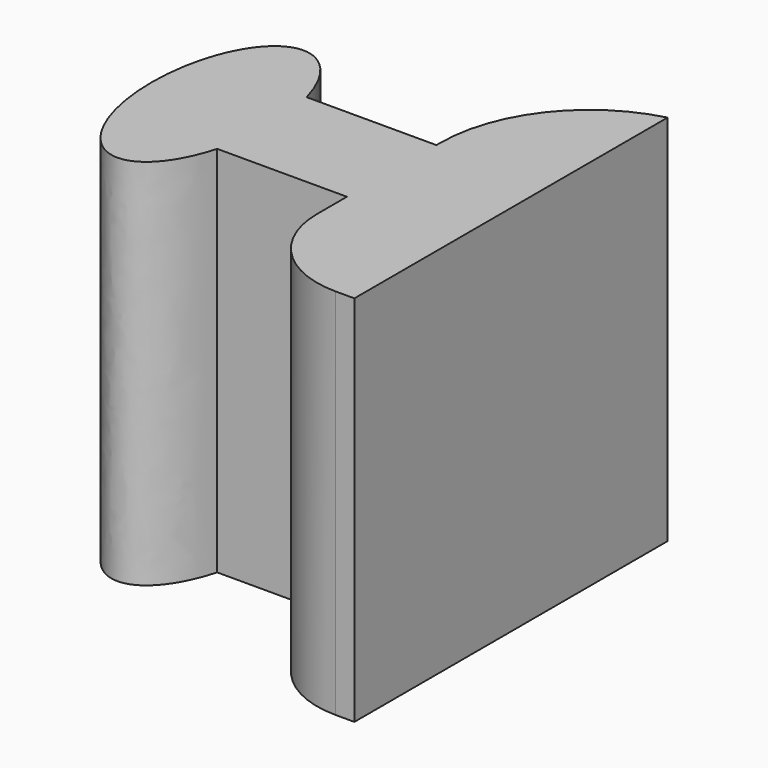
from build123d import *

# Parameters (mm, degrees)
F1_DEPTH    = 10
F2_DEPTH    = 10
F3_T1_DEPTH = 29.364916731
F4_R        = 2.5


# Not quite as in the source:
# - a fillet or chamfer that OpenCascade refuses, or shapes differently, is made with other operations: its cross-section is extruded or revolved along the edge and cut away or added


with BuildPart() as f1:
    # F0 (on Top) → F1 (new body)
    with BuildSketch(Plane.XY):
        with BuildLine():
            Line((0, -5.25), (0, 0))
            Line((0, 0), (0, 5.25))
            Line((0, 5.25), (-3, 5.25))
            Line((-3, 5.25), (-3, 1.25))
            Line((-3, 1.25), (-6.479551384, 1.25))
            add(Edge.make_bspline(
                [(-6.479551384, -1.75), (-6.0631503018, -0.25), (-6.479551384, 1.25)],
                knots=[1.0687204508, 1.0687204508, 1.0687204508, 2.0728722028, 2.0728722028, 2.0728722028], degree=2, weights=[1, 0.8765854438, 1]))
            Line((-6.479551384, -1.75), (-3, -1.75))
            Line((-3, -1.75), (-3, -5.25))
            Line((-3, -5.25), (0, -5.25))
        make_face()
    extrude(amount=F1_DEPTH)

    # F0 (on Top) → F2 (join)
    with BuildSketch(Plane.XY):
        with BuildLine():
            add(Edge.make_bspline(
                [(-6.479551384, -1.75), (-6.0631503018, -0.25), (-6.479551384, 1.25)],
                knots=[1.0687204508, 1.0687204508, 1.0687204508, 2.0728722028, 2.0728722028, 2.0728722028], degree=2, weights=[1, 0.8765854438, 1]))
            add(Edge.make_bspline(
                [(-6.479551384, 1.25), (-7.8097391813, 6.0417303318), (-9.2174427731, 1.3374114859), (-10.6251463649, -3.36690736), (-7.8610982746, -3.36690736)],
                knots=[2.0728722028, 2.0728722028, 2.0728722028, 4.178028755, 4.178028755, 6.2831853072, 6.2831853072, 6.2831853072], degree=2, weights=[1, 0.49533294, 1, 0.49533294, 1]))
            add(Edge.make_bspline(
                [(-7.8610982746, -3.36690736), (-6.9284060337, -3.36690736), (-6.479551384, -1.75)],
                knots=[0, 0, 0, 1.0687204508, 1.0687204508, 1.0687204508], degree=2, weights=[1, 0.8605946365, 1]))
        make_face()
    extrude(amount=F2_DEPTH)

    # F3: fillet of radius 4 on 1 edges, made by hand

    # F3_s2 → F3_t1 (cut)
    with BuildSketch(Plane.XY.offset(-9.6824583655)):
        with BuildLine():
            ThreePointArc((0, 5.25), (-2.1622776602, 3.8265063966), (-3, 1.3770166538))
            Line((-3, 1.3770166538), (-3, 5.25))
            Line((-3, 5.25), (0, 5.25))
        make_face()
    extrude(amount=F3_T1_DEPTH, mode=Mode.SUBTRACT)

    # F4
    f4_edges = [f1.edges().sort_by_distance(p)[0] for p in [
        (-3, -5.25, 5),
    ]]
    fillet(f4_edges, radius=F4_R)


solid = f1.part
